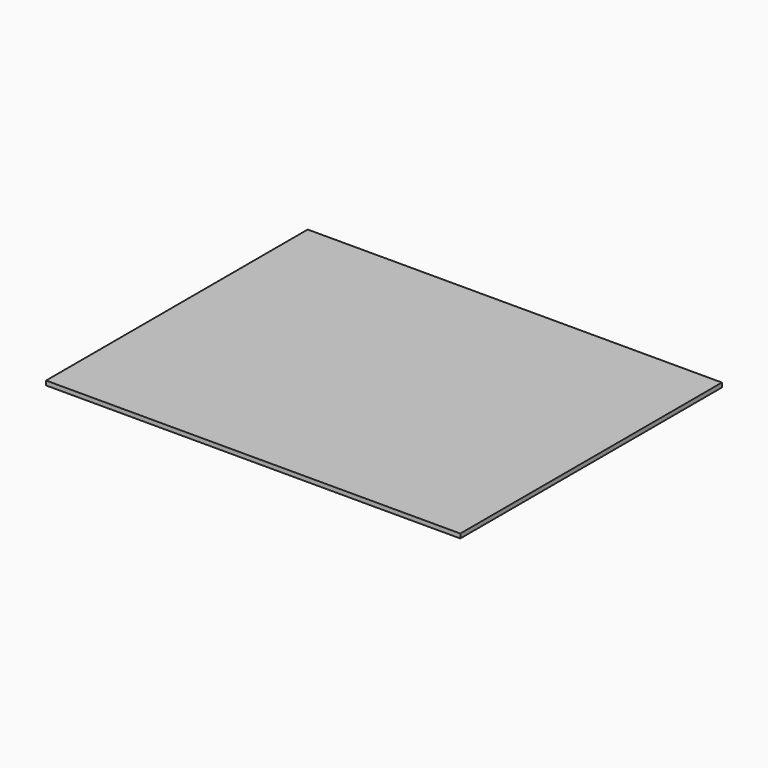
from build123d import *

# Parameters (mm, degrees)
F0_W     = 38
F0_H     = 30
F1_DEPTH = 0.4


# Not quite as in the source:
# - a feature names something its author has since deleted; it is built from what else it names


with BuildPart() as f1:
    # F0 (on Top) → F1 (new body)
    with BuildSketch(Plane.XY):
        Rectangle(F0_W, F0_H)
    extrude(amount=F1_DEPTH)


solid = f1.part
